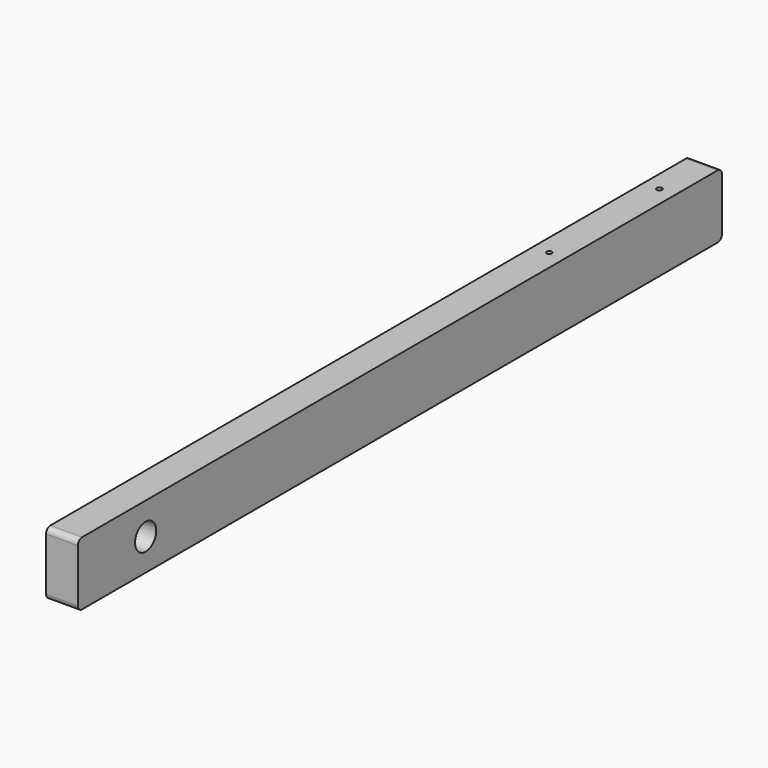
from build123d import *

# Parameters (mm, degrees)
F0_W     = 482.6
F0_H     = 38.1
F0_R     = 7.9375
F1_DEPTH = 9.525
F2_R     = 1.5875
F3_DEPTH = 25.4
F4_R     = 3.175
F5_R     = 3.175


with BuildPart() as f1:
    # F0 (on Right) → F1 (new body, symmetric)
    with BuildSketch(Plane.YZ):
        with Locations((190.5, 0)):
            Rectangle(F0_W, F0_H)
        Circle(F0_R, mode=Mode.SUBTRACT)
    extrude(amount=F1_DEPTH, both=True)

    # F2 (on face) → F3 (cut)
    with BuildSketch(Plane.XY.offset(19.05)):
        with Locations((0, 396.875)):
            Circle(F2_R)
        with Locations((0, 314.325)):
            Circle(F2_R)
    extrude(amount=-F3_DEPTH, mode=Mode.SUBTRACT)

    # F4
    f4_edges = [f1.edges().sort_by_distance(p)[0] for p in [
        (0, 431.8, -19.05),
    ]]
    fillet(f4_edges, radius=F4_R)

    # F5
    f5_edges = [f1.edges().sort_by_distance(p)[0] for p in [
        (0, 431.8, 19.05),
        (0, -50.8, -19.05),
        (0, -50.8, 19.05),
    ]]
    fillet(f5_edges, radius=F5_R)


solid = f1.part
